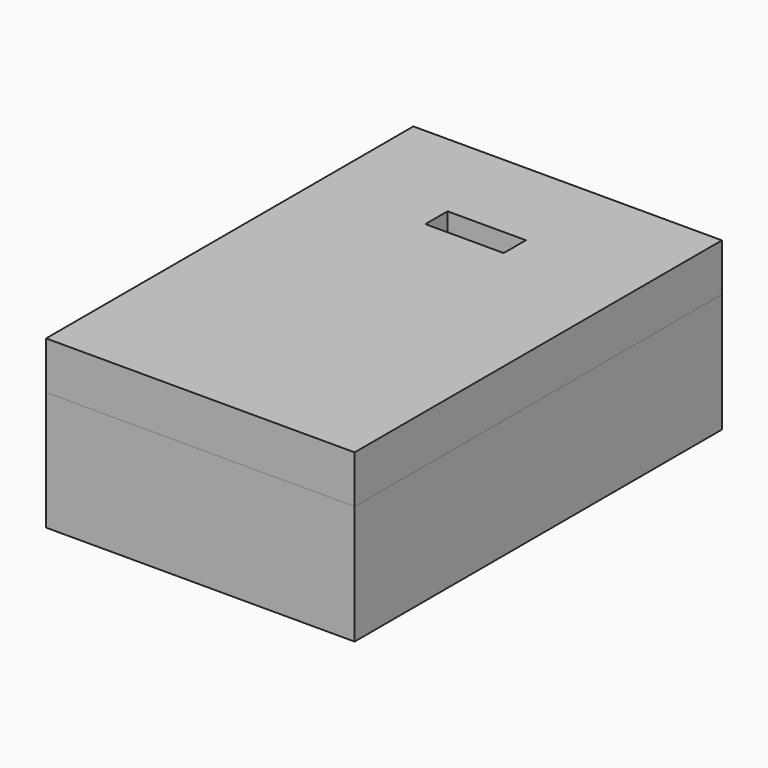
from build123d import *

# Parameters (mm, degrees)
F0_W     = 16.462284606
F0_H     = 24.4974466041
F1_DEPTH = 6.35
F2_W     = 16.462284606
F2_H     = 24.4974466041
F3_DEPTH = 2.54
F4_W     = 4.1798030725
F4_H     = 1.4798403718
F5_DEPTH = 2.54


# Not quite as in the source:
# - a feature names something its author has since deleted; it is built from what else it names


with BuildPart() as f1:
    # F0 (on Top) → F1 (new body)
    with BuildSketch(Plane.XY):
        with Locations((0.2442786936, 0.227171462)):
            Rectangle(F0_W, F0_H)
    extrude(amount=F1_DEPTH)


with BuildPart() as f3:
    # F2 (on face) → F3 (new body)
    with BuildSketch(Plane.XY.offset(6.35)):
        with Locations((0.2442786936, 0.227171462)):
            Rectangle(F2_W, F2_H)
    extrude(amount=F3_DEPTH)

    # F4 (on face) → F5 (cut)
    with BuildSketch(Plane.XY.offset(8.89)):
        with Locations((0.0016469858, 6.6424182151)):
            Rectangle(F4_W, F4_H)
    extrude(amount=-F5_DEPTH, mode=Mode.SUBTRACT)


solid = Compound([f1.part, f3.part])
